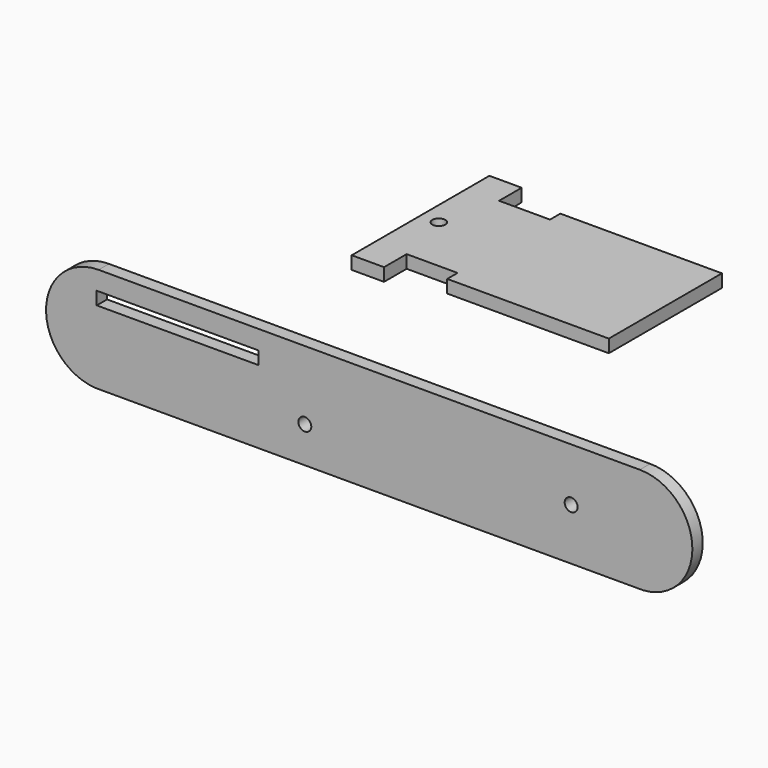
from build123d import *

# Parameters (mm, degrees)
F0_R     = 1.6
F0_W     = 40
F0_H     = 3.2
F1_DEPTH = 3.2
F2_R     = 1.6
F2_W     = 39.3956717427
F2_H     = 28.6
F2_W_2   = 8
F2_H_2   = 7
F3_DEPTH = 3.2


# Not quite as in the source:
# - a feature names something its author has since deleted; it is built from what else it names


with BuildPart() as f1:
    # F0 (on Front) → F1 (new body)
    with BuildSketch(Plane.XZ):
        with BuildLine():
            ThreePointArc((64.2822751435, -12.8260802654), (78.0380924464, -0.2122674413), (65.0326790919, 13.1739197346))
            Line((65.0326790919, 13.1739197346), (-68.9456731455, 13.1739197346))
            ThreePointArc((-68.9456731455, 13.1739197346), (-81.9510814202, 0.5382828094), (-69.6957248565, -12.8260802654))
            Line((-69.6957248565, -12.8260802654), (64.2822751435, -12.8260802654))
        make_face()
        with Locations((-17.8954396397, -3.8823541254)):
            Circle(F0_R, mode=Mode.SUBTRACT)
        with Locations((48.0326790919, 0)):
            Circle(F0_R, mode=Mode.SUBTRACT)
        with Locations((-49.4083422422, 6.8739197346)):
            Rectangle(F0_W, F0_H, mode=Mode.SUBTRACT)
    extrude(amount=F1_DEPTH)


with BuildPart() as f3:
    # F2 (on Top) → F3 (new body)
    with BuildSketch(Plane.XY):
        Polygon((14.0854157835, 50.8921488531), (14.0854157835, 85.8921488531), (-25.9145842165, 85.8921488531), (-25.9145842165, 82.6921488531), (13.4810875262, 82.6921488531), (13.4810875262, 54.0921488531), (-25.9145842165, 54.0921488531), (-25.9145842165, 50.8921488531), align=None)
        Polygon((-25.9145842165, 54.0921488531), (-25.9145842165, 82.6921488531), (-38.5189124738, 82.6921488531), (-46.5189124738, 82.6921488531), (-46.5189124738, 54.0921488531), (-38.5189124738, 54.0921488531), align=None)
        with Locations((-42.0019124738, 68.3921488531)):
            Circle(F2_R, mode=Mode.SUBTRACT)
        with Locations((-6.2167483452, 68.3921488531)):
            Rectangle(F2_W, F2_H)
        with Locations((-42.5189124738, 86.1921488531)):
            Rectangle(F2_W_2, F2_H_2)
        with Locations((-42.5189124738, 50.5921488531)):
            Rectangle(F2_W_2, F2_H_2)
    extrude(amount=F3_DEPTH)


solid = Compound([f1.part, f3.part])
